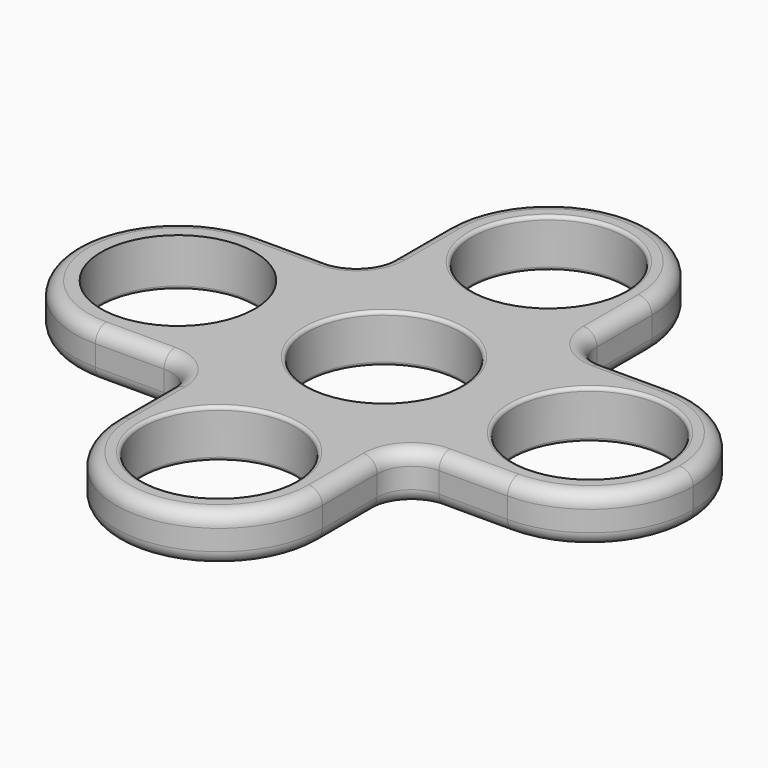
from build123d import *

# Parameters (mm, degrees)
F0_R     = 11.175
F1_DEPTH = 7
F2_R     = 5
F3_R     = 0.5
F4_R     = 2


# Not quite as in the source:
# - a feature names something its author has since deleted; it is built from what else it names


with BuildPart() as f1:
    # F0 (on Top) → F1 (new body)
    with BuildSketch(Plane.XY):
        with BuildLine():
            ThreePointArc((15, -0.7772871268), (14.9848863112, -0.3887741663), (14.9798472864, 0))
            Line((14.9798472864, 0), (11.175, 0))
            ThreePointArc((11.175, 0), (0, -11.175), (-11.175, 0))
            Line((-11.175, 0), (-14.9798472864, 0))
            ThreePointArc((-14.9798472864, 0), (-14.9848863112, -0.3887741663), (-15, -0.7772871268))
            Line((-15, -0.7772871268), (-15, -15))
            Line((-15, -15), (-0.7772871268, -15))
            ThreePointArc((-0.7772871268, -15), (0, -14.9798472864), (0.7772871268, -15))
            Line((0.7772871268, -15), (15, -15))
            Line((15, -15), (15, -0.7772871268))
        make_face()
        with BuildLine():
            ThreePointArc((-0.7772871268, 15), (-10.8779434385, 19.6517135465), (-15, 29.9798472864))
            Line((-15, 29.9798472864), (-15, 15))
            Line((-15, 15), (-0.7772871268, 15))
        make_face()
        with BuildLine():
            ThreePointArc((0.7772871268, 15), (10.8779434385, 19.6517135465), (15, 29.9798472864))
            ThreePointArc((15, 29.9798472864), (0, 44.9798472864), (-15, 29.9798472864))
            ThreePointArc((-15, 29.9798472864), (-10.8779434385, 19.6517135465), (-0.7772871268, 15))
            Line((-0.7772871268, 15), (0, 15))
            Line((0, 15), (0.7772871268, 15))
        make_face()
        with Locations((0, 29.9798472864)):
            Circle(F0_R, mode=Mode.SUBTRACT)
        with BuildLine():
            Line((-15, 0), (-15, 0.7772871268))
            ThreePointArc((-15, 0.7772871268), (-19.6517135465, 10.8779434385), (-29.9798472864, 15))
            ThreePointArc((-29.9798472864, 15), (-44.9798472864, 0), (-29.9798472864, -15))
            ThreePointArc((-29.9798472864, -15), (-19.6517135465, -10.8779434385), (-15, -0.7772871268))
            Line((-15, -0.7772871268), (-15, 0))
        make_face()
        with Locations((-29.9798472864, 0)):
            Circle(F0_R, mode=Mode.SUBTRACT)
        with BuildLine():
            Line((15, 15), (0.7772871268, 15))
            ThreePointArc((0.7772871268, 15), (0, 14.9798472864), (-0.7772871268, 15))
            Line((-0.7772871268, 15), (-15, 15))
            Line((-15, 15), (-15, 0.7772871268))
            ThreePointArc((-15, 0.7772871268), (-14.9848863112, 0.3887741663), (-14.9798472864, 0))
            Line((-14.9798472864, 0), (-11.175, 0))
            ThreePointArc((-11.175, 0), (0, 11.175), (11.175, 0))
            Line((11.175, 0), (14.9798472864, 0))
            ThreePointArc((14.9798472864, 0), (14.9848863112, 0.3887741663), (15, 0.7772871268))
            Line((15, 0.7772871268), (15, 15))
        make_face()
        with BuildLine():
            ThreePointArc((-0.7772871268, 15), (0, 14.9798472864), (0.7772871268, 15))
            Line((0.7772871268, 15), (0, 15))
            Line((0, 15), (-0.7772871268, 15))
        make_face()
        with BuildLine():
            ThreePointArc((-14.9798472864, 0), (-14.9848863112, 0.3887741663), (-15, 0.7772871268))
            Line((-15, 0.7772871268), (-15, 0))
            Line((-15, 0), (-14.9798472864, 0))
        make_face()
        with BuildLine():
            Line((-14.9798472864, 0), (-15, 0))
            Line((-15, 0), (-15, -0.7772871268))
            ThreePointArc((-15, -0.7772871268), (-14.9848863112, -0.3887741663), (-14.9798472864, 0))
        make_face()
        with BuildLine():
            ThreePointArc((29.9798472864, 15), (19.6517135465, 10.8779434385), (15, 0.7772871268))
            Line((15, 0.7772871268), (15, 0))
            Line((15, 0), (15, -0.7772871268))
            ThreePointArc((15, -0.7772871268), (19.6517135465, -10.8779434385), (29.9798472864, -15))
            ThreePointArc((29.9798472864, -15), (40.5864490042, -10.6066017178), (44.9798472864, 0))
            ThreePointArc((44.9798472864, 0), (40.5864490042, 10.6066017178), (29.9798472864, 15))
        make_face()
        with Locations((29.9798472864, 0)):
            Circle(F0_R, mode=Mode.SUBTRACT)
        with BuildLine():
            ThreePointArc((29.9798472864, -15), (19.6517135465, -10.8779434385), (15, -0.7772871268))
            Line((15, -0.7772871268), (15, -15))
            Line((15, -15), (29.9798472864, -15))
        make_face()
        with BuildLine():
            Line((15, -0.7772871268), (15, 0))
            Line((15, 0), (14.9798472864, 0))
            ThreePointArc((14.9798472864, 0), (14.9848863112, -0.3887741663), (15, -0.7772871268))
        make_face()
        with BuildLine():
            Line((15, 0), (15, 0.7772871268))
            ThreePointArc((15, 0.7772871268), (14.9848863112, 0.3887741663), (14.9798472864, 0))
            Line((14.9798472864, 0), (15, 0))
        make_face()
        with BuildLine():
            Line((29.9798472864, 15), (15, 15))
            Line((15, 15), (15, 0.7772871268))
            ThreePointArc((15, 0.7772871268), (19.6517135465, 10.8779434385), (29.9798472864, 15))
        make_face()
        with BuildLine():
            Line((15, 15), (15, 29.9798472864))
            ThreePointArc((15, 29.9798472864), (10.8779434385, 19.6517135465), (0.7772871268, 15))
            Line((0.7772871268, 15), (15, 15))
        make_face()
        with BuildLine():
            Line((0, -15), (-0.7772871268, -15))
            ThreePointArc((-0.7772871268, -15), (-10.8779434385, -19.6517135465), (-15, -29.9798472864))
            ThreePointArc((-15, -29.9798472864), (0, -44.9798472864), (15, -29.9798472864))
            ThreePointArc((15, -29.9798472864), (10.8779434385, -19.6517135465), (0.7772871268, -15))
            Line((0.7772871268, -15), (0, -15))
        make_face()
        with Locations((0, -29.9798472864)):
            Circle(F0_R, mode=Mode.SUBTRACT)
        with BuildLine():
            Line((15, -29.9798472864), (15, -15))
            Line((15, -15), (0.7772871268, -15))
            ThreePointArc((0.7772871268, -15), (10.8779434385, -19.6517135465), (15, -29.9798472864))
        make_face()
        with BuildLine():
            ThreePointArc((0.7772871268, -15), (0, -14.9798472864), (-0.7772871268, -15))
            Line((-0.7772871268, -15), (0, -15))
            Line((0, -15), (0.7772871268, -15))
        make_face()
        with BuildLine():
            Line((-0.7772871268, -15), (-15, -15))
            Line((-15, -15), (-15, -29.9798472864))
            ThreePointArc((-15, -29.9798472864), (-10.8779434385, -19.6517135465), (-0.7772871268, -15))
        make_face()
        with BuildLine():
            ThreePointArc((-15, -0.7772871268), (-19.6517135465, -10.8779434385), (-29.9798472864, -15))
            Line((-29.9798472864, -15), (-15, -15))
            Line((-15, -15), (-15, -0.7772871268))
        make_face()
        with BuildLine():
            Line((-15, 0.7772871268), (-15, 15))
            Line((-15, 15), (-29.9798472864, 15))
            ThreePointArc((-29.9798472864, 15), (-19.6517135465, 10.8779434385), (-15, 0.7772871268))
        make_face()
    extrude(amount=F1_DEPTH)

    # F2
    f2_edges = [f1.edges().sort_by_distance(p)[0] for p in [
        (15, -15, 3.5),
        (-15, -15, 3.5),
        (15, 15, 3.5),
        (-15, 15, 3.5),
    ]]
    fillet(f2_edges, radius=F2_R)

    # F3
    f3_edges = [f1.edges().sort_by_distance(p)[0] for p in [
        (-11.175, 29.979847, 7),
        (11.175, 0, 7),
        (-11.175, 29.979847, 0),
        (11.175, 0, 0),
        (-11.175, -29.979847, 7),
        (-41.154847, 0, 0),
        (18.804847, 0, 0),
        (-11.175, -29.979847, 0),
        (18.804847, 0, 7),
    ]]
    fillet(f3_edges, radius=F3_R)

    # F4
    f4_edges = [f1.edges().sort_by_distance(p)[0] for p in [
        (-16.464466, 16.464466, 0),
        (-15, 20, 3.5),
        (-20, 15, 3.5),
        (-16.464466, 16.464466, 7),
        (-15, 24.989924, 0),
        (-15, 29.979847, 3.5),
        (-15, 24.989924, 7),
        (15, 29.979847, 3.5),
        (0, 44.979847, 0),
        (0, 44.979847, 7),
        (15, 24.989924, 0),
        (15, 20, 3.5),
        (15, 24.989924, 7),
        (16.464466, 16.464466, 0),
        (20, 15, 3.5),
        (16.464466, 16.464466, 7),
        (0, -44.979847, 7),
        (0, -44.979847, 0),
        (15, -24.989924, 0),
        (16.464466, -16.464466, 0),
        (24.989924, -15, 0),
        (-15, -24.989924, 0),
        (44.979847, 0, 0),
        (-16.464466, -16.464466, 0),
        (24.989924, 15, 0),
        (-24.989924, -15, 0),
        (-44.979847, 0, 0),
        (-24.989924, 15, 0),
        (15, -24.989924, 7),
        (16.464466, -16.464466, 7),
        (24.989924, -15, 7),
        (-15, -24.989924, 7),
        (44.979847, 0, 7),
        (-16.464466, -16.464466, 7),
        (24.989924, 15, 7),
        (-24.989924, -15, 7),
        (-44.979847, 0, 7),
        (-24.989924, 15, 7),
    ]]
    fillet(f4_edges, radius=F4_R)


solid = f1.part
